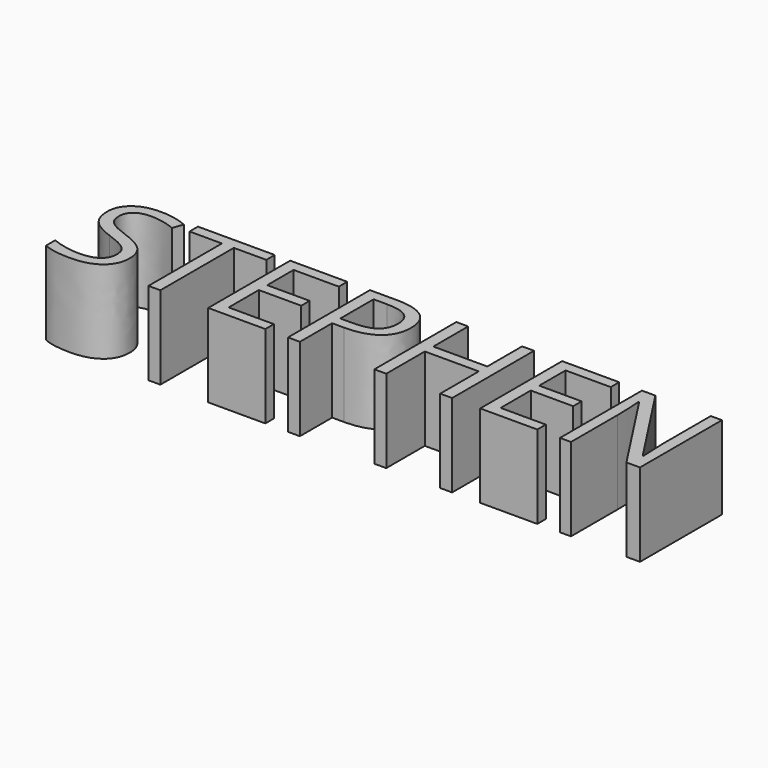
from build123d import *

# Parameters (mm, degrees)
F0_TEXT_SIZE = 73.2055687371
F1_DEPTH     = 42.418


# Not quite as in the source:
# - Text() gives the source's letters only with a copy of the font that has no kerning and outlines rounded to 1/6400 em; it was checked with that copy


with BuildPart() as f1:
    # F0 (on Top) → F1 (new body)
    with BuildSketch(Plane.XY):
        with Locations((-76.4076560736, -2.0855686162)):
            Text('STEPHEN', F0_TEXT_SIZE, font='Open Sans', text_align=(TextAlign.LEFT, TextAlign.BOTTOM))
    extrude(amount=F1_DEPTH)


solid = f1.part
